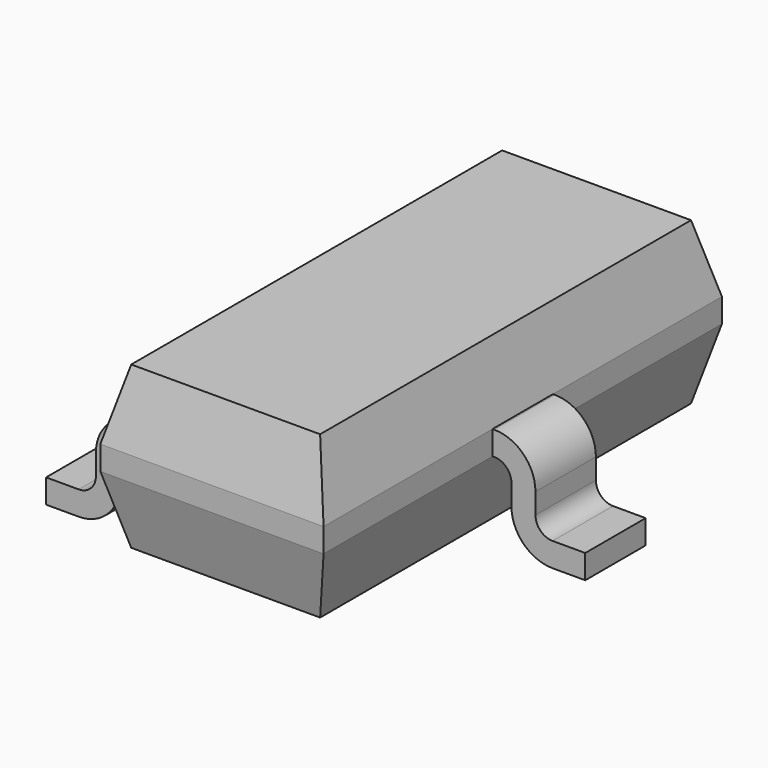
from build123d import *

# Parameters (mm, degrees)
F1_DEPTH    = 0.22
F2_DEPTH    = 1.45
F4_C1_SIZE2 = 0.4
F4_C1_SIZE  = 0.1
F4_C2_SIZE2 = 0.4
F4_C2_SIZE  = 0.1
F4_C3_SIZE2 = 0.4
F4_C3_SIZE  = 0.1
F4_C4_SIZE2 = 0.4
F4_C4_SIZE  = 0.1
F4_C5_SIZE2 = 0.1
F4_C5_SIZE  = 0.4
F4_C6_SIZE2 = 0.4
F4_C6_SIZE  = 0.1
F4_C7_SIZE2 = 0.4
F4_C7_SIZE  = 0.1
F4_C8_SIZE2 = 0.4
F4_C8_SIZE  = 0.1


# Not quite as in the source:
# - a feature of the source that left no trace in its solid (it failed there, or was rolled back) is left out


with BuildPart() as f1:
    # F0 (on Front) → F1 (new body, symmetric)
    with BuildSketch(Plane.XZ):
        Polygon((0.65, -0.07), (0.65, 0.07), (0.4482062359, 0.07), (0.4482062359, 0), (0.4482062359, -0.07), align=None)
        with BuildLine():
            Line((0.66, 0.07), (0.65, 0.07))
            Line((0.65, 0.07), (0.65, -0.07))
            Line((0.65, -0.07), (0.66, -0.07))
            ThreePointArc((0.66, -0.07), (0.7307106781, -0.0992893219), (0.76, -0.17))
            Line((0.76, -0.17), (0.76, -0.29))
            ThreePointArc((0.76, -0.29), (0.8302943725, -0.4597056275), (1, -0.53))
            Line((1, -0.53), (1.19, -0.53))
            Line((1.19, -0.53), (1.19, -0.39))
            Line((1.19, -0.39), (1, -0.39))
            ThreePointArc((1, -0.39), (0.9292893219, -0.3607106781), (0.9, -0.29))
            Line((0.9, -0.29), (0.9, -0.17))
            ThreePointArc((0.9, -0.17), (0.8297056275, -0.0002943725), (0.66, 0.07))
        make_face()
    extrude(amount=F1_DEPTH, both=True)


with BuildPart() as f2:
    # F0 (on Front) → F2 (new body, symmetric)
    with BuildSketch(Plane.XZ):
        Polygon((0.65, 0.47), (-0.65, 0.47), (-0.65, -0.47), (0.65, -0.47), (0.65, -0.07), (0.4482062359, -0.07), (0.4482062359, 0), (0.4482062359, 0.07), (0.65, 0.07), align=None)
        Polygon((0.65, -0.07), (0.65, 0.07), (0.4482062359, 0.07), (0.4482062359, 0), (0.4482062359, -0.07), align=None)
    extrude(amount=F2_DEPTH, both=True)

    # F4: chamfer of 0.4 x 0.1 on 8 edges, made by hand

    # F4_c1
    f4_c1_edges = [f2.edges().sort_by_distance(p)[0] for p in [
        (0, 1.45, 0.47),
    ]]
    f4_c1_side = f2.faces().sort_by_distance((0, 1.448, 0.47))[0]
    chamfer(f4_c1_edges, length=F4_C1_SIZE, length2=F4_C1_SIZE2, reference=f4_c1_side)

    # F4_c2
    f4_c2_edges = [f2.edges().sort_by_distance(p)[0] for p in [
        (-0.65, -0.05, 0.47),
    ]]
    f4_c2_side = f2.faces().sort_by_distance((-0.648, -0.05, 0.47))[0]
    chamfer(f4_c2_edges, length=F4_C2_SIZE, length2=F4_C2_SIZE2, reference=f4_c2_side)

    # F4_c3
    f4_c3_edges = [f2.edges().sort_by_distance(p)[0] for p in [
        (0.05, -1.45, 0.47),
    ]]
    f4_c3_side = f2.faces().sort_by_distance((0.05, -1.448, 0.47))[0]
    chamfer(f4_c3_edges, length=F4_C3_SIZE, length2=F4_C3_SIZE2, reference=f4_c3_side)

    # F4_c4
    f4_c4_edges = [f2.edges().sort_by_distance(p)[0] for p in [
        (0.65, 0, 0.47),
    ]]
    f4_c4_side = f2.faces().sort_by_distance((0.648, 0, 0.47))[0]
    chamfer(f4_c4_edges, length=F4_C4_SIZE, length2=F4_C4_SIZE2, reference=f4_c4_side)

    # F4_c5
    f4_c5_edges = [f2.edges().sort_by_distance(p)[0] for p in [
        (0.65, 0, -0.47),
    ]]
    f4_c5_side = f2.faces().sort_by_distance((0.65, 0, -0.468))[0]
    chamfer(f4_c5_edges, length=F4_C5_SIZE, length2=F4_C5_SIZE2, reference=f4_c5_side)

    # F4_c6
    f4_c6_edges = [f2.edges().sort_by_distance(p)[0] for p in [
        (-0.65, 0, -0.47),
    ]]
    f4_c6_side = f2.faces().sort_by_distance((-0.648, 0, -0.47))[0]
    chamfer(f4_c6_edges, length=F4_C6_SIZE, length2=F4_C6_SIZE2, reference=f4_c6_side)

    # F4_c7
    f4_c7_edges = [f2.edges().sort_by_distance(p)[0] for p in [
        (0, 1.45, -0.47),
    ]]
    f4_c7_side = f2.faces().sort_by_distance((0, 1.448, -0.47))[0]
    chamfer(f4_c7_edges, length=F4_C7_SIZE, length2=F4_C7_SIZE2, reference=f4_c7_side)

    # F4_c8
    f4_c8_edges = [f2.edges().sort_by_distance(p)[0] for p in [
        (0, -1.45, -0.47),
    ]]
    f4_c8_side = f2.faces().sort_by_distance((0, -1.448, -0.47))[0]
    chamfer(f4_c8_edges, length=F4_C8_SIZE, length2=F4_C8_SIZE2, reference=f4_c8_side)


with BuildPart() as f3_1:
    # F3: instance of F1
    add(f1.part.mirror(Plane.YZ))


with BuildPart() as f3_1_1:
    # F6: moved
    add(f3_1.part.moved(Location((0, 0.95, 0))))


with BuildPart() as f7_1:
    # F7: instance of F3_1
    add(f3_1_1.part.mirror(Plane.XZ))


solid = Compound([f1.part, f2.part, f3_1_1.part, f7_1.part])
